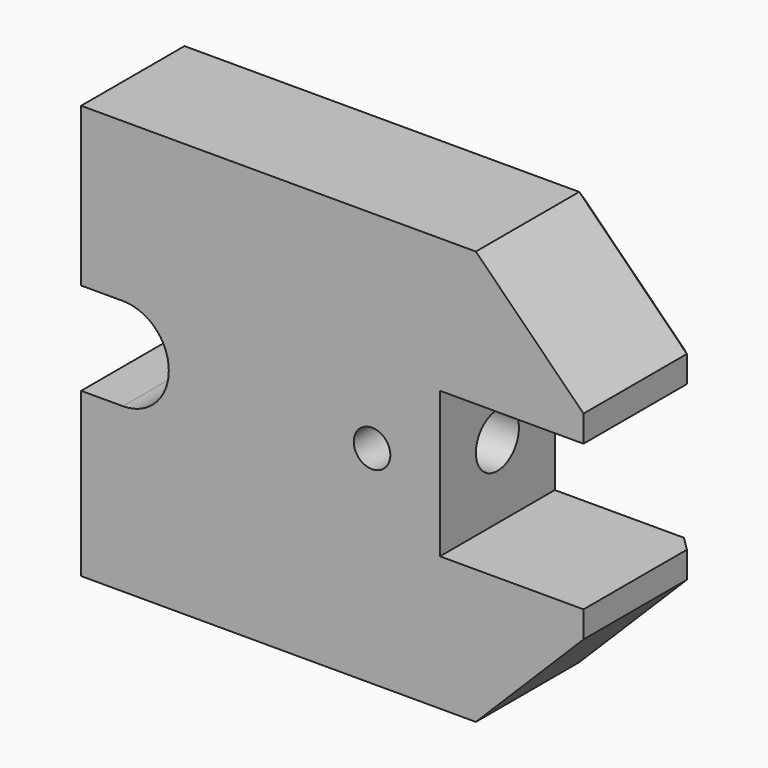
from build123d import *

# Parameters (mm, degrees)
F1_DEPTH    = 25.4
F2_SIZE     = 2.54
F3_T1_DEPTH = 120.8411218415
F4_SIZE     = 2.54
F5_W        = 15.5079813242
F5_H        = 16.3934864104
F6_DEPTH    = 25.4
F7_R        = 8.128
F9_D        = 9.525
F9_DEPTH    = 19.05
F9_TIP      = 2.8615986981
F11_D       = 6.477
F11_DEPTH   = 14.2748
F11_TIP     = 1.9458871147


# Not quite as in the source:
# - a fillet or chamfer that OpenCascade refuses, or shapes differently, is made with other operations: its cross-section is extruded or revolved along the edge and cut away or added


with BuildPart() as f1:
    # F0 (on Front) → F1 (new body)
    with BuildSketch(Plane.XZ):
        Polygon((-88.9, 0), (0, 0), (0, 23.7338524312), (-25.4, 23.7338524312), (-25.4, 49.53), (0, 49.53), (0, 73.279), (-88.9, 73.279), align=None)
    extrude(amount=F1_DEPTH)

    # F2
    f2_edges = [f1.edges().sort_by_distance(p)[0] for p in [
        (-44.45, 0, 73.279),
        (0, 0, 61.4045),
        (-88.9, 0, 36.6395),
        (-44.45, 0, 0),
        (0, 0, 11.866926),
    ]]
    chamfer(f2_edges, length=F2_SIZE)

    # F3: chamfer of 19.05 on 2 edges, made by hand

    # F3_s2 → F3_t1 (cut)
    with BuildSketch(Plane.XZ.offset(-46.4505609208)):
        Polygon((-19.05, 73.279), (0, 54.229), (0, 73.279), align=None)
        Polygon((-19.05, 0), (0, 19.05), (0, 0), align=None)
    extrude(amount=F3_T1_DEPTH, mode=Mode.SUBTRACT)

    # F4
    f4_edges = [f1.edges().sort_by_distance(p)[0] for p in [
        (-9.525, 0, 63.754),
        (-9.525, 0, 9.525),
    ]]
    chamfer(f4_edges, length=F4_SIZE)

    # F5 (on face) → F6 (cut)
    with BuildSketch(Plane.XZ.offset(25.4)):
        with Locations((-81.1460093379, 37.0688531548)):
            Rectangle(F5_W, F5_H)
    extrude(amount=-F6_DEPTH, mode=Mode.SUBTRACT)

    # F7
    f7_edges = [f1.edges().sort_by_distance(p)[0] for p in [
        (-73.392019, -12.7, 45.265596),
        (-73.392019, -12.7, 28.87211),
    ]]
    fillet(f7_edges, radius=F7_R)

    # F9
    with Locations(Plane.YZ.offset(-25.4)):
        with Locations((-12.7, 36.6319262156)):
            Hole(F9_D / 2, depth=F9_DEPTH)
            with Locations((0, 0, -(F9_DEPTH + F9_TIP / 2))):  # 118° drill point
                Cone(0, F9_D / 2, F9_TIP, mode=Mode.SUBTRACT)

    # F11
    with Locations(Plane.XZ.offset(25.4)):
        with Locations((-37.4242216349, 36.6319262156)):
            Hole(F11_D / 2, depth=F11_DEPTH)
            with Locations((0, 0, -(F11_DEPTH + F11_TIP / 2))):  # 118° drill point
                Cone(0, F11_D / 2, F11_TIP, mode=Mode.SUBTRACT)


solid = f1.part
